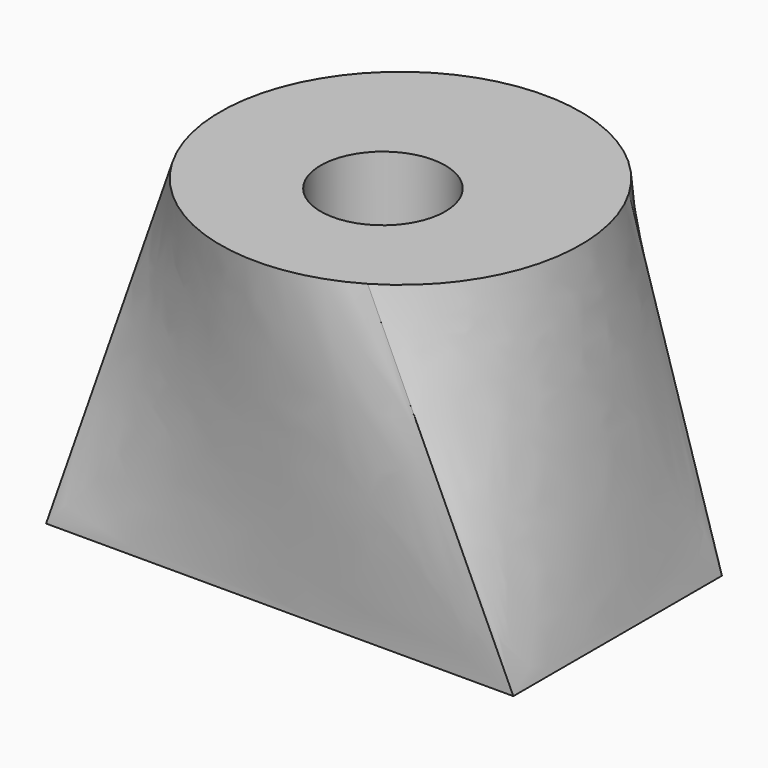
from build123d import *

# Parameters (mm, degrees)
F0_W     = 43.1823767722
F0_H     = 24.0973075852
F4_R     = 5.7616257058
F5_DEPTH = 30


# Not quite as in the source:
# - the arcs of a loft's sections are written as splines that run evenly, so that the points pair up as in the source's solid


with BuildPart() as f3:
    # F2 (on offset) → F3 section 0
    with BuildSketch(Plane.XY.offset(30)):
        with BuildLine():
            add(Edge.make_bspline(
                [(-14.3525502898, -6.4258121346), (-13.7994999926, -7.3651843545), (-13.1539455701, -8.2500639934), (-11.7025735307, -9.8769193643), (-10.8967918018, -10.618854869), (-9.1559237309, -11.9313020315), (-8.2208804354, -12.5017812365), (-6.2574169169, -13.4493835823), (-5.2290452443, -13.8264832918), (-3.1184410799, -14.3728249941), (-2.036260777, -14.5420534776), (0.1403746989, -14.6661389313), (1.2347760501, -14.6209928331), (3.3937959567, -14.3180535037), (4.4583611261, -14.0602677631), (6.5167955393, -13.3419454391), (7.5106138842, -12.8814266176), (8.449986104, -12.3283763204)],
                knots=[0, 0, 0, 0, 0.125, 0.125, 0.25, 0.25, 0.375, 0.375, 0.5, 0.5, 0.625, 0.625, 0.75, 0.75, 0.875, 0.875, 1, 1, 1, 1], degree=3))
            add(Edge.make_bspline(
                [(8.449986104, -12.3283763204), (9.3893583239, -11.7753260232), (10.2742379628, -11.1297716007), (11.9010933337, -9.6783995613), (12.6430288384, -8.8726178324), (13.9554760009, -7.1317497615), (14.5259552059, -6.196706466), (15.4735575517, -4.2332429475), (15.8506572612, -3.2048712749), (16.3969989635, -1.0942671105), (16.566227447, -0.0120868075), (16.6903129007, 2.1645486683), (16.6451668025, 3.2589500195), (16.3422274731, 5.4179699262), (16.0844417325, 6.4825350955), (15.3661194086, 8.5409695087), (14.905600587, 9.5347878536), (14.3525502898, 10.4741600735)],
                knots=[0, 0, 0, 0, 0.125, 0.125, 0.25, 0.25, 0.375, 0.375, 0.5, 0.5, 0.625, 0.625, 0.75, 0.75, 0.875, 0.875, 1, 1, 1, 1], degree=3))
            add(Edge.make_bspline(
                [(14.3525502898, 10.4741600735), (13.7994999926, 11.4135322933), (13.1539455701, 12.2984119322), (11.7025735307, 13.9252673031), (10.8967918018, 14.6672028078), (9.1559237309, 15.9796499703), (8.2208804354, 16.5501291753), (6.2574169169, 17.4977315211), (5.2290452443, 17.8748312306), (3.1184410799, 18.4211729329), (2.036260777, 18.5904014164), (-0.1403746989, 18.7144868701), (-1.2347760501, 18.6693407719), (-3.3937959567, 18.3664014425), (-4.4583611261, 18.108615702), (-6.5167955393, 17.390293378), (-7.5106138842, 16.9297745564), (-8.449986104, 16.3767242592)],
                knots=[0, 0, 0, 0, 0.125, 0.125, 0.25, 0.25, 0.375, 0.375, 0.5, 0.5, 0.625, 0.625, 0.75, 0.75, 0.875, 0.875, 1, 1, 1, 1], degree=3))
            add(Edge.make_bspline(
                [(-8.449986104, 16.3767242592), (-9.3893583239, 15.823673962), (-10.2742379628, 15.1781195395), (-11.9010933337, 13.7267475001), (-12.6430288384, 12.9209657712), (-13.9554760009, 11.1800977003), (-14.5259552059, 10.2450544049), (-15.4735575517, 8.2815908863), (-15.8506572612, 7.2532192137), (-16.3969989635, 5.1426150493), (-16.566227447, 4.0604347464), (-16.6903129007, 1.8837992705), (-16.6451668025, 0.7893979193), (-16.3422274731, -1.3696219873), (-16.0844417325, -2.4341871567), (-15.3661194086, -4.4926215699), (-14.905600587, -5.4864399148), (-14.3525502898, -6.4258121346)],
                knots=[0, 0, 0, 0, 0.125, 0.125, 0.25, 0.25, 0.375, 0.375, 0.5, 0.5, 0.625, 0.625, 0.75, 0.75, 0.875, 0.875, 1, 1, 1, 1], degree=3))
        make_face()
    # F0 (on Top) → F3 section 1
    with BuildSketch(Plane.XY):
        with Locations((-0.6747245789, 0.963892322)):
            Rectangle(F0_W, F0_H)
    loft(ruled=True)

    # F4 (on face) → F5 (cut)
    with BuildSketch(Plane.XY.offset(30)):
        Circle(F4_R)
    extrude(amount=-F5_DEPTH, mode=Mode.SUBTRACT)


solid = f3.part
